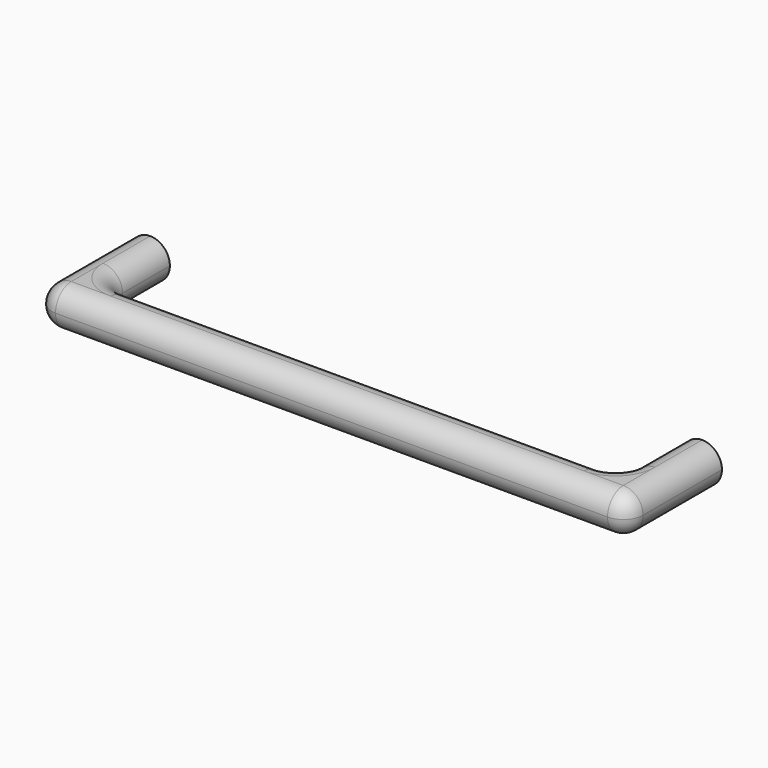
from build123d import *

# Parameters (mm, degrees)
F0_W     = 190.5
F0_H     = 12.7
F1_DEPTH = 38.1
F2_W     = 165.1
F2_H     = 25.4
F3_DEPTH = 12.701
F4_R     = 6.34999


# Not quite as in the source:
# - a fillet or chamfer is up to 0.001 mm smaller than in the source, because OpenCascade refuses the exact size


with BuildPart() as f1:
    # F0 (on Front) → F1 (new body)
    with BuildSketch(Plane.XZ):
        Rectangle(F0_W, F0_H)
    extrude(amount=F1_DEPTH)

    # F2 (on face) → F3 (cut, through all)
    with BuildSketch(Plane.XY.offset(6.35)):
        with Locations((0, -12.7)):
            Rectangle(F2_W, F2_H)
    extrude(amount=-F3_DEPTH, mode=Mode.SUBTRACT)

    # F4 (radius 6.35 in the source; OpenCascade refuses exactly that, so slightly less here)
    f4_edges = [f1.edges().sort_by_distance(p)[0] for p in [
        (-95.25, -38.1, 0),
        (-82.55, -25.4, 0),
        (95.25, -38.1, 0),
        (82.55, -25.4, 0),
        (0, -38.1, 6.35),
        (0, -25.4, 6.35),
        (0, -38.1, -6.35),
        (0, -25.4, -6.35),
        (-82.55, -12.7, -6.35),
        (-95.25, -19.05, -6.35),
        (82.55, -12.7, -6.35),
        (95.25, -19.05, -6.35),
        (95.25, -19.05, 6.35),
        (-82.55, -12.7, 6.35),
        (-95.25, -19.05, 6.35),
        (82.55, -12.7, 6.35),
    ]]
    fillet(f4_edges, radius=F4_R)


solid = f1.part
